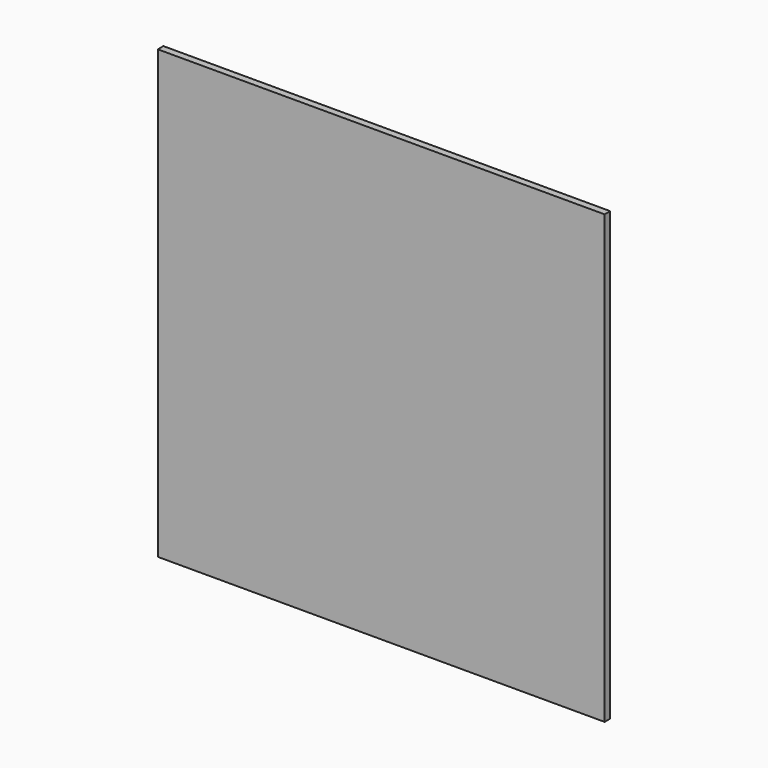
from build123d import *

# Parameters (mm, degrees)
F0_W     = 1219.2
F0_H     = 1219.2
F1_DEPTH = 19.05


# Not quite as in the source:
# - a feature names something its author has since deleted; it is built from what else it names


with BuildPart() as f1:
    # F0 (on Front) → F1 (new body)
    with BuildSketch(Plane.XZ):
        Rectangle(F0_W, F0_H)
    extrude(amount=F1_DEPTH)


solid = f1.part
